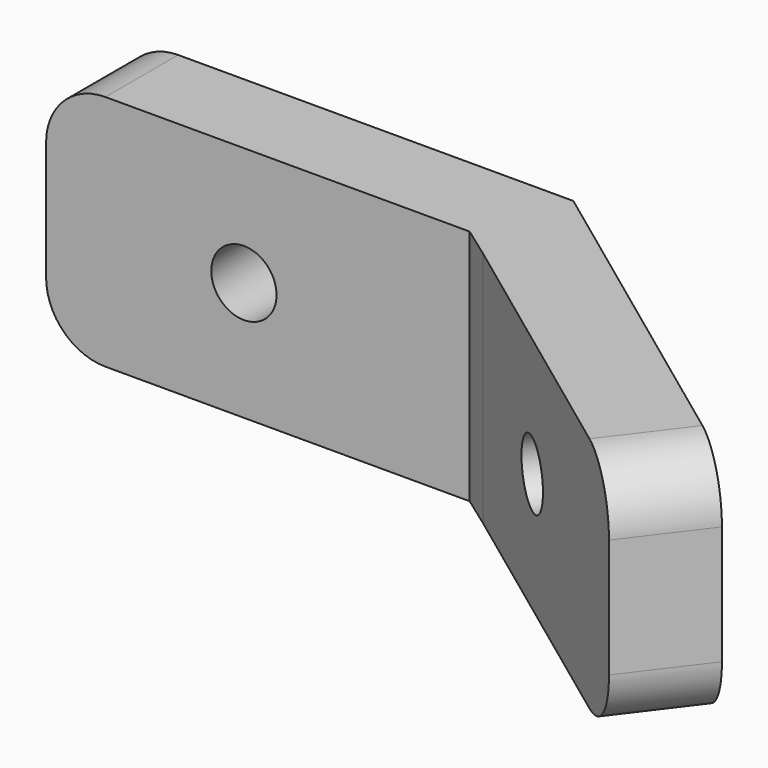
from build123d import *

# Parameters (mm, degrees)
F1_DEPTH = 12
F2_R     = 1.65
F3_DEPTH = 27.5381246112
F4_R     = 1.65
F5_DEPTH = 17.26183437
F6_R     = 3


# Not quite as in the source:
# - a feature names something its author has since deleted; it is built from what else it names


with BuildPart() as f1:
    # F0 (on Top) → F1 (new body)
    with BuildSketch(Plane.XY):
        Polygon((-22.9726818199, 5.7206649829), (-22.9726818199, 1.1206649829), (-1.5669824788, 1.1206649829), (0.8286588168, 1.1206649829), (2.734780124, 3.6984730734), (0, 5.7206649829), align=None)
        Polygon((2.734780124, 3.6984730734), (0.8286588168, 1.1206649829), (0, 0), (15.6067412389, -11.5401693871), (18.3798691562, -7.870052011), align=None)
        Polygon((0.8286588168, 1.1206649829), (-1.5669824788, 1.1206649829), (0, 0), align=None)
    extrude(amount=F1_DEPTH)

    # F2 (on face) → F3 (cut, through all)
    with BuildSketch(Plane(origin=(2.734780124, 3.6984730734, 0), x_dir=(-0.8040591029, 0.5945493747, 0), z_dir=(0.5945493747, 0.8040591029, 0))):
        with Locations((-7.5987822114, 6)):
            Circle(F2_R)
    extrude(amount=-F3_DEPTH, mode=Mode.SUBTRACT)

    # F4 (on face) → F5 (cut, through all)
    with BuildSketch(Plane(origin=(0, 5.7206649829, 0), x_dir=(-1, 0, 0), z_dir=(0, 1, 0))):
        with Locations((12.9726818199, 6)):
            Circle(F4_R)
    extrude(amount=-F5_DEPTH, mode=Mode.SUBTRACT)

    # F6
    f6_edges = [f1.edges().sort_by_distance(p)[0] for p in [
        (-22.972682, 3.420665, 12),
        (-22.972682, 3.420665, 0),
        (16.993305, -9.705111, 0),
        (16.993305, -9.705111, 12),
    ]]
    fillet(f6_edges, radius=F6_R)


solid = f1.part
